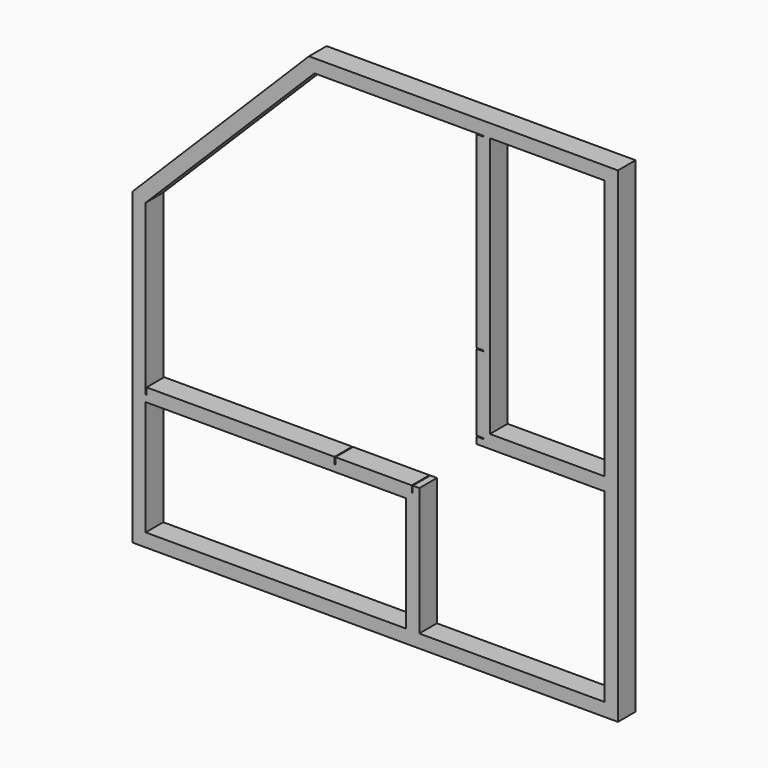
from build123d import *

# Parameters (mm, degrees)
F1_DEPTH = 25


# Not quite as in the source:
# - ends of sketch curves that miss each other by under 0.0002 mm in the source are joined


with BuildPart() as f1:
    # F0 (on Front) → F1 (new body)
    with BuildSketch(Plane.XZ):
        Polygon((-275, 53.7867965644), (-275, -275), (275, -275), (275, 275), (-68.7867965644, 275), (-68.7867965644, 260), (115, 260), (115, 267.5000010639), (130, 267.5000010639), (130, 260), (260, 260), (260, -35), (267.5, -35), (267.5, -50), (260, -50), (260, -260), (50, -260), (50, -267.5), (35, -267.5), (35, -260), (-260, -260), (-260, -130), (-267.5, -130), (-267.5, -115), (-260, -115), (-260, 68.7867965644), (-268.7268512791, 60.0599452853), align=None)
        Polygon((-275, 68.7867965644), (-275, 53.7867965644), (-268.7268512791, 60.0599452853), (-260, 68.7867965644), align=None)
        Polygon((-275, 75), (-275, 68.7867965644), (-260, 68.7867965644), align=None)
        Polygon((-68.7867965644, 260), (-68.7867965644, 275), (-75, 275), align=None)
        Polygon((-79.3933982822, 270.6066017178), (-275, 75), (-260, 68.7867965644), (-68.7867965644, 260), align=None)
        Polygon((-68.7867965644, 260), (-75, 275), (-79.3933982822, 270.6066017178), align=None)
        Polygon((-260, -122.5), (-260, -115), (-267.5, -115), (-267.5, -130), (-260, -130), (35, -130), (35, -260), (35, -267.5), (50, -267.5), (50, -260), (50, -115), (42.5, -115), (42.5, -122.5), (41.5, -122.5), (41.5, -115), (39.3933982822, -115), (-44.3324317381, -115), (-45, -115), (-45, -122.5), (-46, -122.5), (-46, -115), (-258.5857843554, -115), (-259, -115), (-259, -115.414213564), (-259, -122.5), align=None)
        Polygon((115, 267.5000010639), (115, 260), (122.5, 260), (122.5, 259), (115.414213564, 259), (115, 259), (115, 258.5857864337), (115, 46), (122.5, 46), (122.5, 45), (115, 45), (115, -41.5), (122.5, -41.5), (122.5, -42.5), (115, -42.5), (115, -50), (260, -50), (267.5, -50), (267.5, -35), (260, -35), (130, -35), (130, 260), (130, 267.5000010639), align=None)
    extrude(amount=F1_DEPTH)


solid = f1.part
